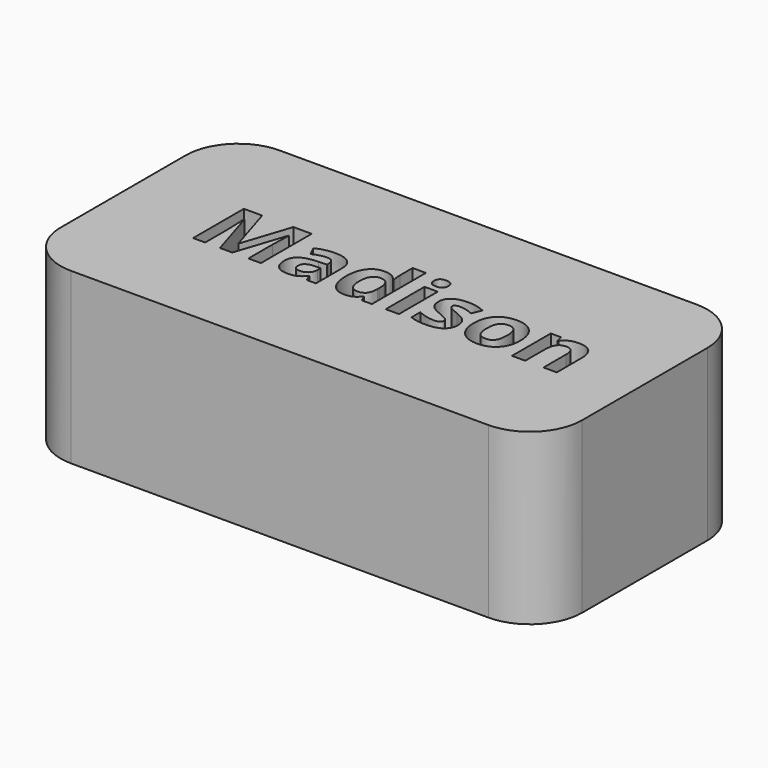
from build123d import *

# Parameters (mm, degrees)
F0_W         = 50.8
F0_H         = 16.51
F1_DEPTH     = 25.4
F2_TEXT_SIZE = 8.6520695024
F3_DEPTH     = 25.4
F4_R         = 5.08


# Not quite as in the source:
# - Text() gives the source's letters only with a copy of the font that has no kerning and outlines rounded to 1/6400 em; it was checked with that copy


with BuildPart() as f1:
    # F0 (on Front) → F1 (new body)
    with BuildSketch(Plane.XZ):
        with Locations((25.4, 8.255)):
            Rectangle(F0_W, F0_H)
    extrude(amount=F1_DEPTH)

    # F2 (on face) → F3 (cut)
    with BuildSketch(Plane.XY.offset(16.51)):
        with Locations((8.1762066111, -15.3790516779)):
            Text('Madison', F2_TEXT_SIZE, font='Open Sans', font_style=FontStyle.BOLD, text_align=(TextAlign.LEFT, TextAlign.BOTTOM))
    extrude(amount=-F3_DEPTH, mode=Mode.SUBTRACT)

    # F4
    f4_edges = [f1.edges().sort_by_distance(p)[0] for p in [
        (0, -25.4, 8.255),
        (50.8, -25.4, 8.255),
        (50.8, 0, 8.255),
        (0, 0, 8.255),
    ]]
    fillet(f4_edges, radius=F4_R)


solid = f1.part
